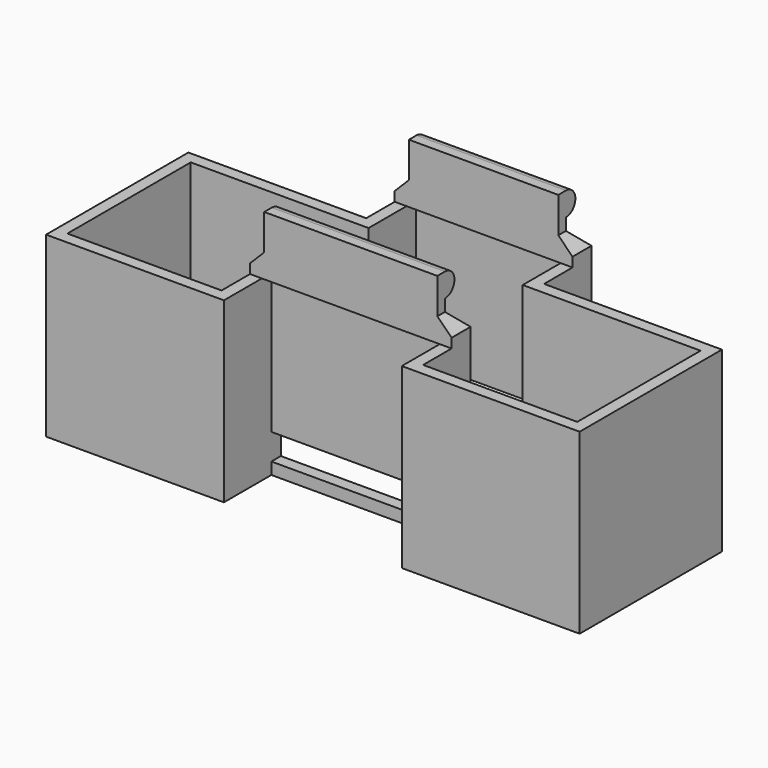
from build123d import *

# Parameters (mm, degrees)
F3_DEPTH  = 15
F4_W      = 1
F4_H      = 1
F4_W_2    = 15
F4_W_3    = 13
F5_DEPTH  = 2
F6_SIZE   = 1.2
F7_DEPTH  = 3
F8_W      = 14.6
F8_H      = 2
F9_W      = 12.6
F9_H      = 2
F10_DEPTH = 1
F11_R     = 0.99999
F12_W     = 15
F12_H     = 2.2
F13_W     = 13
F13_H     = 2.2
F14_DEPTH = 1


# Not quite as in the source:
# - a fillet or chamfer is up to 0.001 mm smaller than in the source, because OpenCascade refuses the exact size


with BuildPart() as f3:
    # F2 (on Top) → F3 (new body)
    with BuildSketch(Plane.XY):
        Polygon((-39.3307432532, 0), (-24.3307432532, 0), (-24.3307432532, 5), (-24.3307432532, 6), (-25.3307432532, 6), (-25.3307432532, 1), (-38.3307432532, 1), (-38.3307432532, 14), (-25.3307432532, 14), (-24.3307432532, 14), (-24.3307432532, 15), (-39.3307432532, 15), align=None)
        Polygon((-24.3307432532, 6), (-24.3307432532, 5), (-9.3307432532, 5), (-9.3307432532, 6), (-10.3307432532, 6), (-23.3307432532, 6), align=None)
        Polygon((-9.3307432532, 6), (-9.3307432532, 5), (-9.3307432532, 0), (5.6692567468, 0), (5.6692567468, 15), (-9.3307432532, 15), (-9.3307432532, 14), (-8.3307432532, 14), (4.6692567468, 14), (4.6692567468, 1), (-8.3307432532, 1), (-8.3307432532, 6), align=None)
        Polygon((-24.3307432532, 20), (-24.3307432532, 15), (-24.3307432532, 14), (-23.3307432532, 14), (-23.3307432532, 19), (-10.3307432532, 19), (-10.3307432532, 14), (-9.3307432532, 14), (-9.3307432532, 15), (-9.3307432532, 20), align=None)
    extrude(amount=F3_DEPTH)

    # F4 (on face) → F5 (join)
    with BuildSketch(Plane.XY.offset(15)):
        Polygon((-8.3307432532, 6), (-25.3307432532, 6), (-25.3307432532, 5), (-24.3307432532, 5), (-9.3307432532, 5), (-8.3307432532, 5), align=None)
        with Locations((-8.8307432532, 4.5)):
            Rectangle(F4_W, F4_H)
        with Locations((-16.8307432532, 4.5)):
            Rectangle(F4_W_2, F4_H)
        with Locations((-24.8307432532, 4.5)):
            Rectangle(F4_W, F4_H)
        Polygon((-24.3307432532, 19), (-23.3307432532, 19), (-10.3307432532, 19), (-9.3307432532, 19), (-9.3307432532, 20), (-24.3307432532, 20), align=None)
        with Locations((-23.8307432532, 18.5)):
            Rectangle(F4_W, F4_H)
        with Locations((-16.8307432532, 18.5)):
            Rectangle(F4_W_3, F4_H)
        with Locations((-9.8307432532, 18.5)):
            Rectangle(F4_W, F4_H)
    extrude(amount=F5_DEPTH)

    # F6
    f6_edges = [f3.edges().sort_by_distance(p)[0] for p in [
        (-16.830743, 6, 17),
        (-25.330743, 5, 17),
        (-8.330743, 5, 17),
        (-16.830743, 20, 17),
        (-24.330743, 19, 17),
        (-9.330743, 19, 17),
    ]]
    chamfer(f6_edges, length=F6_SIZE)

    # F7 (add): faces of the model
    f7_faces = [f3.faces().sort_by_distance(p)[0] for p in [
        (-16.8307432532, 4.4, 17),
        (-16.8307432532, 18.4, 17),
    ]]
    extrude(f7_faces, amount=F7_DEPTH)

    # F8 (on face) + F9 (on face) → F10 (join)
    with BuildSketch(Plane(origin=(0, 4.8, 0), x_dir=(-1, 0, 0), z_dir=(0, 1, 0))):
        with Locations((16.8307432532, 19)):
            Rectangle(F8_W, F8_H)
    with BuildSketch(Plane(origin=(0, 18.8, 0), x_dir=(-1, 0, 0), z_dir=(0, 1, 0))):
        with Locations((16.8307432532, 19)):
            Rectangle(F9_W, F9_H)
    extrude(amount=F10_DEPTH)

    # F11 (radius 1 in the source; OpenCascade refuses exactly that, so slightly less here)
    f11_edges = [f3.edges().sort_by_distance(p)[0] for p in [
        (-16.830743, 5.8, 20),
        (-16.830743, 5.8, 18),
        (-16.830743, 19.8, 20),
        (-16.830743, 19.8, 18),
    ]]
    fillet(f11_edges, radius=F11_R)

    # F12 (on face) + F13 (on face) → F14 (cut, through all)
    with BuildSketch(Plane.XZ.offset(-5)):
        with Locations((-16.8307432532, 2.1)):
            Rectangle(F12_W, F12_H)
    with BuildSketch(Plane.XZ.offset(-19)):
        with Locations((-16.8307432532, 2.1)):
            Rectangle(F13_W, F13_H)
    extrude(amount=-F14_DEPTH, mode=Mode.SUBTRACT)


solid = f3.part
